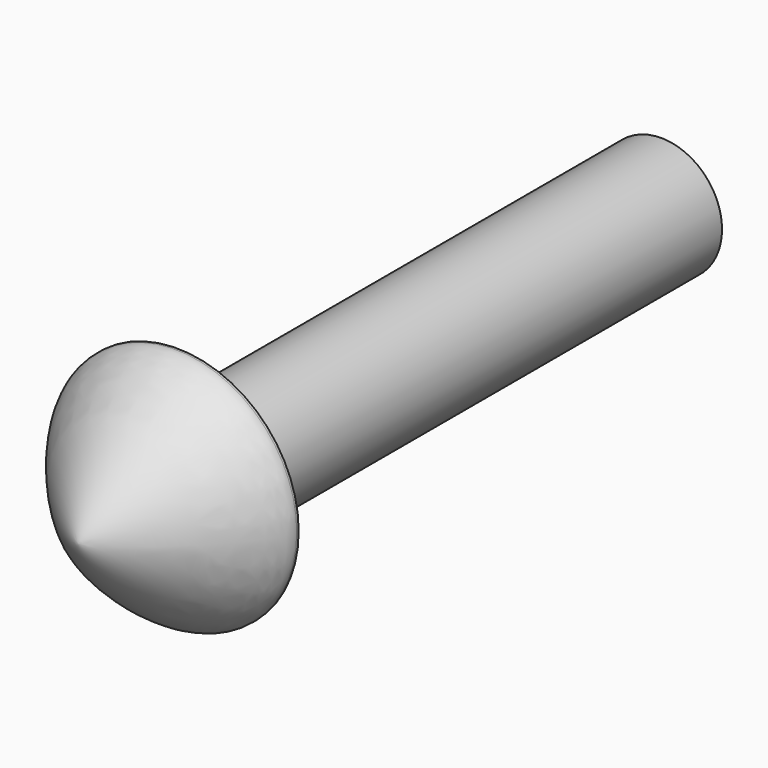
from build123d import *

# Parameters (mm, degrees)
F0_R     = 12.7
F1_DEPTH = 76.2
F3_R     = 12.7
F3_R_2   = 6.35
F4_DEPTH = 63.246
F5_R     = 2.1129626077
F6_DEPTH = 12.7


# Not quite as in the source:
# - a fillet or chamfer that OpenCascade refuses, or shapes differently, is made with other operations: its cross-section is extruded or revolved along the edge and cut away or added


with BuildPart() as f1:
    # F0 (on Front) → F1 (new body)
    with BuildSketch(Plane.XZ):
        Circle(F0_R)
    extrude(amount=F1_DEPTH)

    # F2: fillet of radius 12.7 on 1 edges, made by hand

    # F2_s1 → F2_t2 (revolve, cut)
    with BuildSketch(Plane.XY):
        with BuildLine():
            add(Edge.make_bspline(
                [(12.7, -63.5), (12.7, -76.2), (0, -76.2)],
                knots=[0, 0, 0, 1, 1, 1], degree=2, weights=[1, 0.1764705882, 1]))
            Line((0, -76.2), (12.7, -76.2))
            Line((12.7, -76.2), (12.7, -63.5))
        make_face()
    revolve(axis=Axis((0, -76.2, 0), (0, -1, 0)), mode=Mode.SUBTRACT)

    # F3 (on face) → F4 (cut)
    with BuildSketch(Plane(origin=(0, 0, 0), x_dir=(-1, 0, 0), z_dir=(0, 1, 0))):
        Circle(F3_R)
        Circle(F3_R_2, mode=Mode.SUBTRACT)
    extrude(amount=-F4_DEPTH, mode=Mode.SUBTRACT)

    # F5 (on face) → F6 (cut)
    with BuildSketch(Plane(origin=(0, 0, 0), x_dir=(-1, 0, 0), z_dir=(0, 1, 0))):
        Circle(F5_R)
    extrude(amount=-F6_DEPTH, mode=Mode.SUBTRACT)


solid = f1.part
